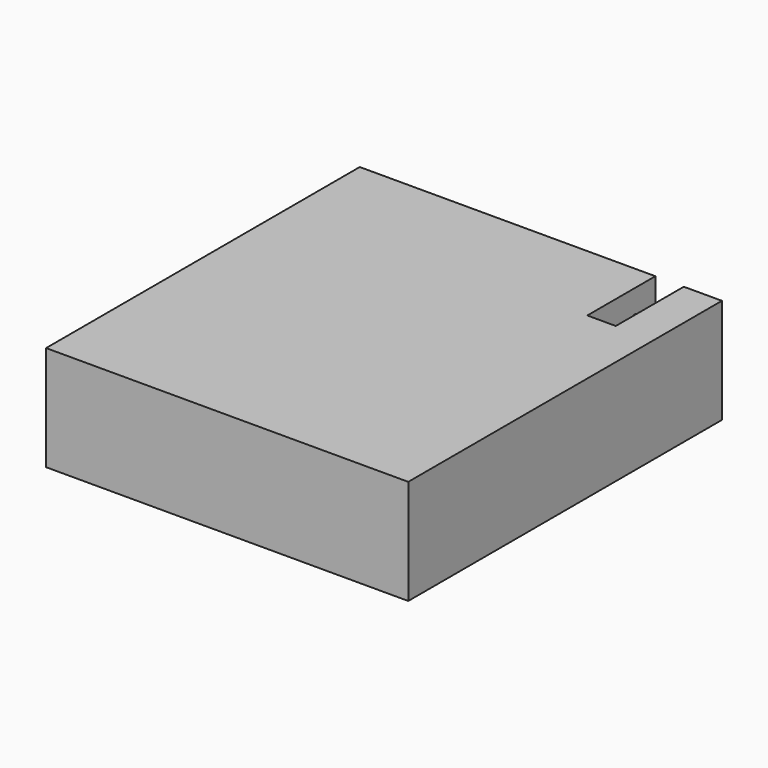
from build123d import *

# Parameters (mm, degrees)
F0_W     = 87.7047851682
F0_H     = 94.9464440346
F1_DEPTH = 25.4
F4_W     = 6.8936049938
F4_H     = 20.5912292004
F5_DEPTH = 10.6445495039
F6_R     = 1.3068757952
F7_DEPTH = 71.5821401606


# Not quite as in the source:
# - the program builds the solid bodies; features that only make, move or delete a surface that nothing else refers to are left out


with BuildPart() as f1:
    # F0 (on Top) → F1 (new body)
    with BuildSketch(Plane.XY):
        with Locations((7.1410946548, -16.8972313404)):
            Rectangle(F0_W, F0_H)
    extrude(amount=F1_DEPTH)

    # F4 (on face) → F5 (cut)
    with BuildSketch(Plane.XY.offset(25.4)):
        with Locations((38.3166447282, 20.2803760767)):
            Rectangle(F4_W, F4_H)
    extrude(amount=-F5_DEPTH, mode=Mode.SUBTRACT)

    # F6 (on face) → F7 (cut, through all)
    with BuildSketch(Plane.YZ.offset(34.8698422313)):
        with Locations((24.3584793061, 18.4984076768)):
            Circle(F6_R)
    extrude(amount=-F7_DEPTH, mode=Mode.SUBTRACT)


solid = f1.part
